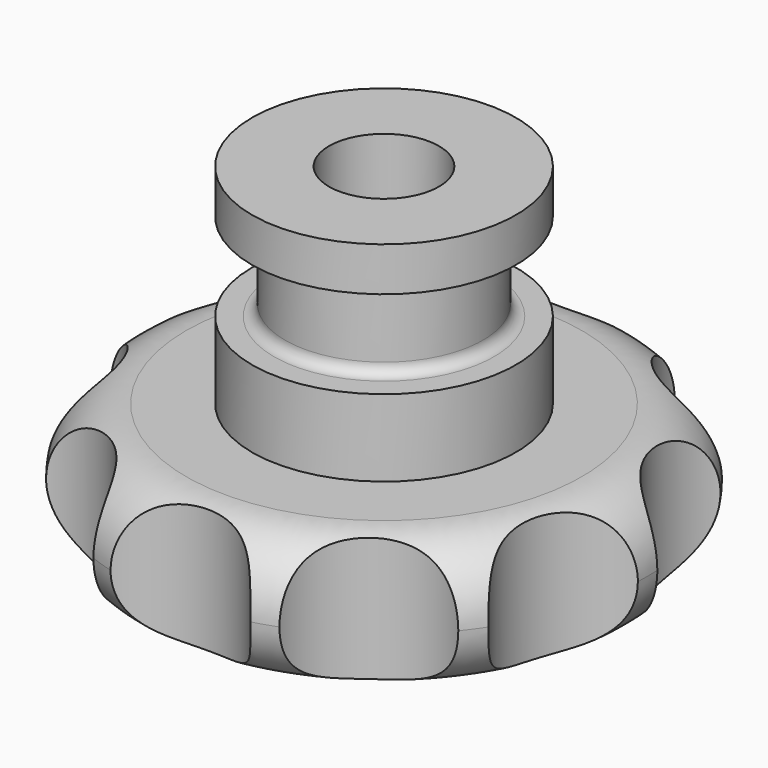
from build123d import *

# Parameters (mm, degrees)
F2_R     = 2.99999
F3_R     = 4
F4_DEPTH = 25
F5_R     = 0.5


# Not quite as in the source:
# - a fillet or chamfer is up to 0.001 mm smaller than in the source, because OpenCascade refuses the exact size


with BuildPart() as f1:
    # F0 (on Front) → F1 (revolve)
    with BuildSketch(Plane.XZ):
        Polygon((-2.5, 4), (-2.5, 15.5), (-6, 15.5), (-6, 13.5), (-4.5, 13.5), (-4.5, 9.5), (-6, 9.5), (-6, 6), (-12, 6), (-12, 0), (0, 0), (0, 4), align=None)
    revolve(axis=Axis((0, 0, 2), (0, 0, -1)))

    # F2 (radius 3 in the source; OpenCascade refuses exactly that, so slightly less here)
    f2_edges = [f1.edges().sort_by_distance(p)[0] for p in [
        (12, 0, 6),
        (12, 0, 0),
    ]]
    fillet(f2_edges, radius=F2_R)

    # F3 (on face) → F4 (cut)
    with BuildSketch(Plane.XY.offset(6)):
        with Locations((0, 14)):
            Circle(F3_R)
        with Locations((8.2289935321, 11.3262379212)):
            Circle(F3_R)
        with Locations((13.3147912281, 4.3262379212)):
            Circle(F3_R)
        with Locations((13.3147912281, -4.3262379212)):
            Circle(F3_R)
        with Locations((8.2289935321, -11.3262379212)):
            Circle(F3_R)
        with Locations((0, -14)):
            Circle(F3_R)
        with Locations((-8.2289935321, -11.3262379212)):
            Circle(F3_R)
        with Locations((-13.3147912281, -4.3262379212)):
            Circle(F3_R)
        with Locations((-13.3147912281, 4.3262379212)):
            Circle(F3_R)
        with Locations((-8.2289935321, 11.3262379212)):
            Circle(F3_R)
    extrude(amount=-F4_DEPTH, mode=Mode.SUBTRACT)

    # F5
    f5_edges = [f1.edges().sort_by_distance(p)[0] for p in [
        (4.5, 0, 13.5),
        (4.5, 0, 9.5),
    ]]
    fillet(f5_edges, radius=F5_R)


solid = f1.part
